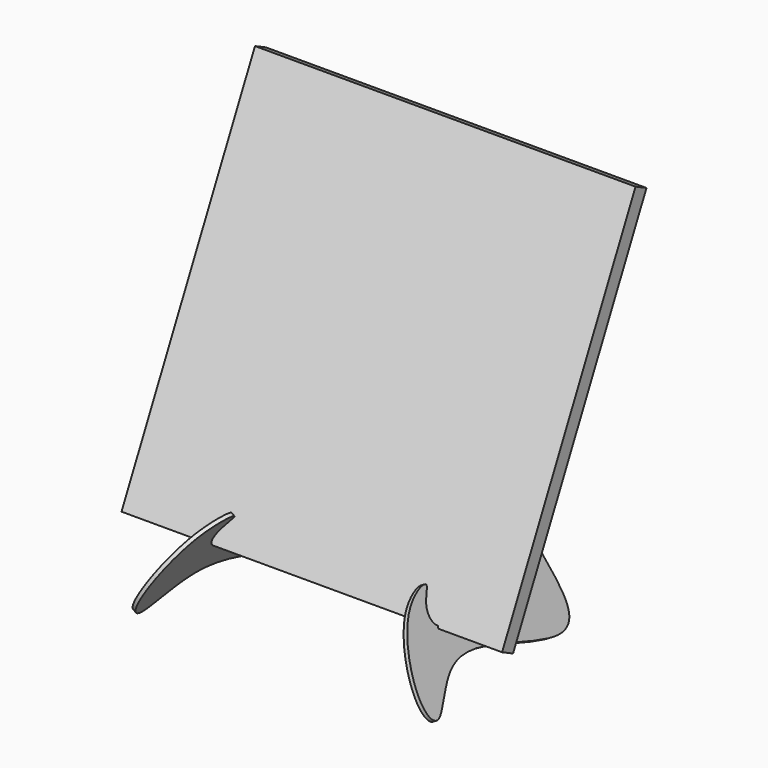
from build123d import *

# Parameters (mm, degrees)
F0_W      = 300
F0_H      = 300
F1_DEPTH  = 12
F4_ANGLE  = 15
F6_DEPTH  = 3
F7_ANGLE  = 30
F12_DEPTH = 25
F14_ANGLE = 11


with BuildPart() as f1:
    # F0 (on Front) → F1 (new body)
    with BuildSketch(Plane.XZ):
        Rectangle(F0_W, F0_H)
    extrude(amount=F1_DEPTH)


with BuildPart() as f1_1:
    # F4: moved
    add(f1.part.rotate(Axis((0, 0, -150), (-1, 0, 0)), F4_ANGLE))


with BuildPart() as f6:
    # F5 (on Right) → F6 (new body)
    with BuildSketch(Plane.YZ):
        with BuildLine():
            add(Edge.make_bspline(
                [(60.7347326074, 58.6497646588), (65.6291503102, 64.3809417215), (112.7549649515, 59.1414982), (125.7698219839, 6.0946642527), (100.2685365269, -42.9806504404), (66.7173481961, -88.0603520299), (80.482443725, -150.2556119456), (82.3170938127, -185.3394703369), (59.5887628827, -195.1120265624), (-0.2961348855, -169.9664897865), (-52.7910904024, -159.4803897301), (-83.0987121994, -198.959207047), (-97.7296314308, -174.5817355433), (-75.2784892157, -118.0291005801), (-30.9743280967, -112.0473833671), (-50.8156300077, -125.425093018), (-50.0728721412, -144.3242769935), (-21.9076684505, -146.6485126347), (7.7911480216, -161.8251289885), (48.1439631386, -88.3778279245), (63.6455387115, -25.6548930409), (75.219802068, 30.0031442519), (56.8256436632, 54.0723701141), (60.7347326074, 58.6497646588)],
                knots=[0, 0, 0, 0, 0.0494011202, 0.101993407, 0.1581479503, 0.2143379667, 0.2745009271, 0.3169661428, 0.3489241504, 0.4102027059, 0.4657991965, 0.5119585705, 0.5421505134, 0.6011496618, 0.6407536587, 0.668156957, 0.6969114266, 0.7351174713, 0.7742208697, 0.8388665096, 0.9036072288, 0.9605441577, 1, 1, 1, 1], degree=3))
        make_face()
    extrude(amount=F6_DEPTH)


with BuildPart() as f6_1:
    # F7: moved
    add(f6.part.rotate(Axis((-150, -5.7955549577, -148.4470857294), (0, 0.9659258263, -0.2588190451)), F7_ANGLE))


with BuildPart() as f8_1:
    # F8: instance of F6
    add(f6_1.part.mirror(Plane.YZ))


with BuildPart() as f8_1_1:
    # F9: moved
    add(f8_1.part.moved(Location((136, 0, 0))))

    # F11 (on face) → F12 (cut)
    with BuildSketch(Plane(origin=(19.2593904406, 2.8779161797, 10.7405294024), x_dir=(0.1130223122, -0.9915912341, 0.0630300046), z_dir=(-0.8660254038, -0.1294095226, -0.4829629131))):
        Polygon((-106.9518650504, -119.5554200444), (-105.575258298, -124.570195613), (-64.7203114356, -115.0897722004), (-65.8948737558, -110.0281120678), align=None)
    extrude(amount=-F12_DEPTH, mode=Mode.SUBTRACT)


with BuildPart() as f1_2:
    # F13: moved
    add(f1_1.part.moved(Location((59, -54, -68))))


with BuildPart() as f1_3:
    # F14: moved
    add(f1_2.part.rotate(Axis((59, -65.5911099155, -214.8941714588), (-1, 0, 0)), F14_ANGLE))


solid = Compound([f6_1.part, f8_1_1.part, f1_3.part])
